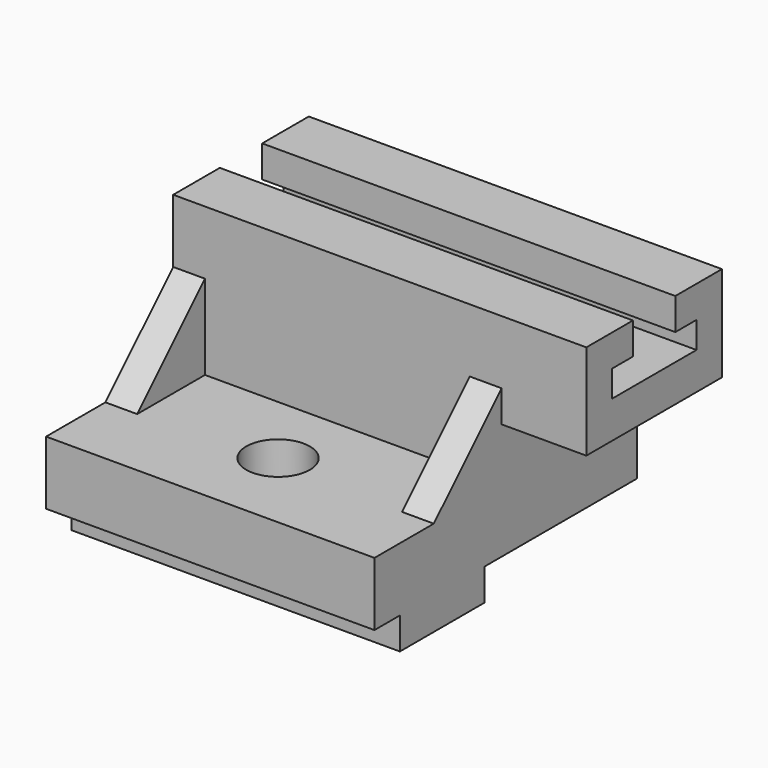
from build123d import *

# Parameters (mm, degrees)
F0_W      = 98.425
F0_H      = 19.05
F1_DEPTH  = 98.425
F2_W      = 98.425
F2_H      = 31.75
F3_DEPTH  = 9.525
F5_DEPTH  = 58.928
F6_W      = 98.425
F6_H      = 50.8
F7_DEPTH  = 44.45
F8_W      = 98.425
F8_H      = 15.875
F9_DEPTH  = 17.4625
F10_W     = 7.9375
F10_H     = 7.9375
F11_DEPTH = 104.394
F13_DEPTH = 25.4
F14_W     = 9.525
F14_H     = 25.4
F15_DEPTH = 31.242
F17_DEPTH = 25.4
F19_DEPTH = 39.878
F21_DEPTH = 25.4


with BuildPart() as f1:
    # F0 (on Front) → F1 (new body)
    with BuildSketch(Plane.XZ):
        with Locations((16.241223073, -7.6058536083)):
            Rectangle(F0_W, F0_H)
    extrude(amount=F1_DEPTH)

    # F2 (on face) → F3 (join)
    with BuildSketch(Plane(origin=(0, 0, -17.1308536083), x_dir=(1, 0, 0), z_dir=(0, 0, -1))):
        with Locations((16.241223073, 73.025)):
            Rectangle(F2_W, F2_H)
    extrude(amount=F3_DEPTH)

    # F4 (on face) → F5 (cut)
    with BuildSketch(Plane.XY.offset(1.9191463917)):
        with BuildLine():
            ThreePointArc((16.241223073, -82.55), (22.9764151638, -79.7601920908), (25.766223073, -73.025))
            ThreePointArc((25.766223073, -73.025), (9.5060309822, -66.2898079092), (16.241223073, -82.55))
        make_face()
    extrude(amount=-F5_DEPTH, mode=Mode.SUBTRACT)

    # F6 (on face) → F7 (join)
    with BuildSketch(Plane.XY.offset(1.9191463917)):
        with Locations((16.241223073, -25.4)):
            Rectangle(F6_W, F6_H)
    extrude(amount=F7_DEPTH)

    # F8 (on face) → F9 (cut)
    with BuildSketch(Plane.XY.offset(46.3691463917)):
        with Locations((16.241223073, -25.4)):
            Rectangle(F8_W, F8_H)
    extrude(amount=-F9_DEPTH, mode=Mode.SUBTRACT)

    # F10 (on face) → F11 (cut)
    with BuildSketch(Plane(origin=(-32.971276927, 0, 0), x_dir=(0, -1, 0), z_dir=(-1, 0, 0))):
        with Locations((13.49375, 32.8753963917)):
            Rectangle(F10_W, F10_H)
        with Locations((37.30625, 32.8753963917)):
            Rectangle(F10_W, F10_H)
    extrude(amount=-F11_DEPTH, mode=Mode.SUBTRACT)

    # F12 (on face) → F13 (join)
    with BuildSketch(Plane.YZ.offset(65.453723073)):
        Polygon((-33.3375, 46.3691463917), (-50.8, 46.3691463917), (-50.8, 17.7941463917), (0, 17.7941463917), (0, 46.3691463917), (-17.4625, 46.3691463917), (-17.4625, 36.8441463917), (-9.525, 36.8441463917), (-9.525, 28.9066463917), (-41.275, 28.9066463917), (-41.275, 36.8441463917), (-33.3375, 36.8441463917), align=None)
    extrude(amount=F13_DEPTH)

    # F14 (on face) → F15 (join)
    with BuildSketch(Plane.XZ.offset(50.8)):
        with Locations((-28.208776927, 14.6191463917)):
            Rectangle(F14_W, F14_H)
    extrude(amount=F15_DEPTH)

    # F16 (on face) → F17 (cut)
    with BuildSketch(Plane.YZ.offset(-23.446276927)):
        Polygon((-76.2, 1.9191463917), (-50.8, 27.3191463917), (-82.042, 27.3191463917), (-82.042, 1.9191463917), align=None)
    extrude(amount=-F17_DEPTH, mode=Mode.SUBTRACT)

    # F18 (on face) → F19 (join)
    with BuildSketch(Plane.XZ.offset(50.8)):
        Polygon((55.928723073, 1.9191463917), (65.453723073, 1.9191463917), (65.453723073, 17.7941463917), (65.453723073, 27.3191463917), (55.928723073, 27.3191463917), align=None)
    extrude(amount=F19_DEPTH)

    # F20 (on face) → F21 (cut)
    with BuildSketch(Plane(origin=(55.928723073, 0, 0), x_dir=(0, -1, 0), z_dir=(-1, 0, 0))):
        Polygon((90.678, 27.3191463917), (50.8, 27.3191463917), (76.2, 1.9191463917), (90.678, 1.9191463917), align=None)
    extrude(amount=-F21_DEPTH, mode=Mode.SUBTRACT)


solid = f1.part
